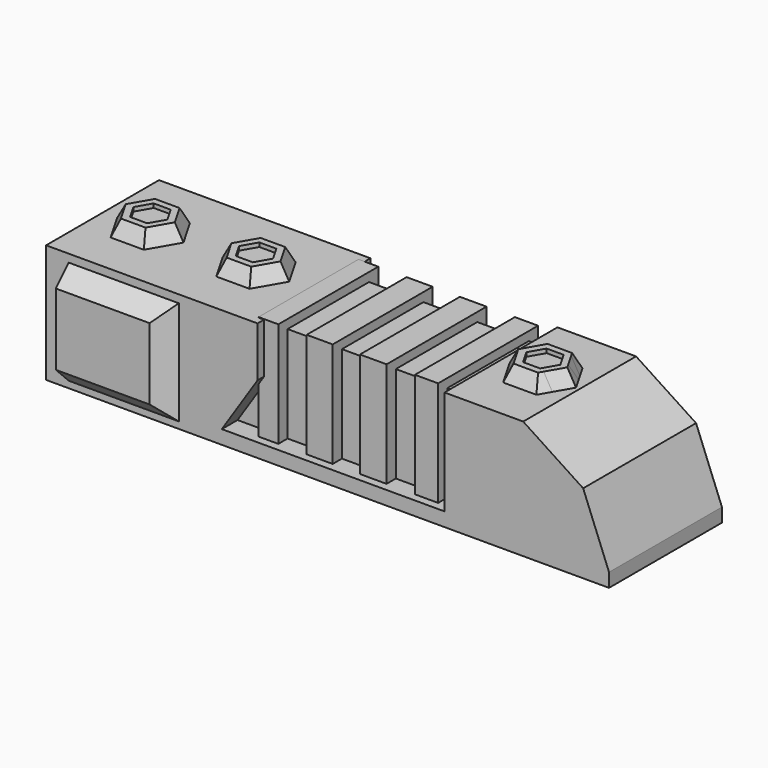
from build123d import *

# Parameters (mm, degrees)
F1_DEPTH      = 15.494
F2_W          = 63.7689922005
F2_H          = 21.1620870978
F3_DEPTH      = 11.176
F4_W          = 5.0933659077
F4_H          = 23.1081098318
F4_W_2        = 5.8479374275
F4_W_3        = 5.7101263665
F4_W_4        = 4.3384544551
F5_DEPTH      = 13.716
F7_DEPTH      = 26.289
F8_T4_DEPTH   = 30.6763762067
F8_T11_DEPTH  = 30.6763762067
F8_T18_DEPTH  = 30.6763762067
F8_T25_DEPTH  = 30.6763762067
F8_T32_DEPTH  = 30.6763762067
F8_T39_DEPTH  = 30.6763762067
F8_T46_DEPTH  = 30.6763762067
F8_T53_DEPTH  = 30.6763762067
F8_T60_DEPTH  = 30.6763762067
F8_T67_DEPTH  = 30.6763762067
F8_T74_DEPTH  = 30.6763762067
F8_T81_DEPTH  = 30.6763762067
F8_T89_DEPTH  = 30.6763762067
F8_T94_DEPTH  = 30.6763762067
F8_T103_DEPTH = 30.6763762067
F8_T109_DEPTH = 30.6763762067
F8_T118_DEPTH = 30.6763762067
F8_T123_DEPTH = 30.6763762067
F8_T131_DEPTH = 30.6763762067
F8_T137_DEPTH = 30.6763762067
F8_T146_DEPTH = 30.6763762067
F8_T152_DEPTH = 30.6763762067
F8_T161_DEPTH = 30.6763762067
F8_T167_DEPTH = 30.6763762067
F8_T175_DEPTH = 30.6763762067
F8_T180_DEPTH = 30.6763762067
F8_T189_DEPTH = 30.6763762067
F8_T195_DEPTH = 30.6763762067
F8_T203_DEPTH = 30.6763762067
F8_T208_DEPTH = 30.6763762067
F8_T216_DEPTH = 30.6763762067
F8_T222_DEPTH = 30.6763762067
F8_T230_DEPTH = 30.6763762067
F8_T236_DEPTH = 30.6763762067
F8_T244_DEPTH = 30.6763762067
F8_T249_DEPTH = 30.6763762067
F10_DEPTH     = 51.054
F11_W         = 19.0685391426
F11_H         = 12.6749693882
F12_DEPTH     = 19.05
F13_T4_DEPTH  = 19.0685391426
F13_T9_DEPTH  = 12.6749693882
F13_T14_DEPTH = 19.0685391426
F13_T19_DEPTH = 19.0685391426
F13_T24_DEPTH = 12.6749693882
F13_T29_DEPTH = 19.0685391426
F13_T35_DEPTH = 32.1326887215
F13_T40_DEPTH = 25.739118967
F13_T49_DEPTH = 32.1326887215
F13_T54_DEPTH = 25.739118967
F13_T63_DEPTH = 32.1326887215
F13_T68_DEPTH = 25.739118967
F13_T77_DEPTH = 32.1326887215
F13_T82_DEPTH = 25.739118967
F14_T4_DEPTH  = 30.6763762067
F14_T11_DEPTH = 30.6763762067
F14_T18_DEPTH = 30.6763762067
F14_T25_DEPTH = 30.6763762067
F14_T32_DEPTH = 30.6763762067
F14_T39_DEPTH = 30.6763762067
F15_DEPTH     = 25.4


# Not quite as in the source:
# - a fillet or chamfer that OpenCascade refuses, or shapes differently, is made with other operations: its cross-section is extruded or revolved along the edge and cut away or added


with BuildPart() as f1:
    # F0 (on Front) → F1 (new body, symmetric)
    with BuildSketch(Plane.XZ):
        Polygon((-61.5085139871, 22.9873508215), (-61.5085139871, 0), (-22.9227617383, 0), (-15.0710064918, 11.9948992506), (-15.0710064918, 22.9873508215), align=None)
        Polygon((-22.9227617383, 0), (-61.5085139871, 0), (-61.5085139871, -3.0355965719), (62.1004961431, -3.0355965719), (62.1004961431, 0), (25.9824357927, 0), align=None)
        Polygon((25.9824357927, 22.9873508215), (25.9824357927, 0), (62.1004961431, 0), (56.4225864728, 14.368809454), (43.256290257, 22.9873508215), align=None)
    extrude(amount=F1_DEPTH, both=True)

    # F2 (on Front) → F3 (join, symmetric)
    with BuildSketch(Plane.XZ):
        with Locations((1.4678305015, 10.5810435489)):
            Rectangle(F2_W, F2_H)
    extrude(amount=F3_DEPTH, both=True)

    # F4 (on Front) → F5 (join, symmetric)
    with BuildSketch(Plane.XZ):
        with Locations((20.6055901945, 11.5540549159)):
            Rectangle(F4_W, F4_H)
        with Locations((8.9097167365, 11.5540549159)):
            Rectangle(F4_W_2, F4_H)
        with Locations((-2.8550631832, 11.5540549159)):
            Rectangle(F4_W_3, F4_H)
        with Locations((-14.1045767814, 11.5540549159)):
            Rectangle(F4_W_4, F4_H)
    extrude(amount=F5_DEPTH, both=True)

    # F6 (on Top) → F7 (join)
    with BuildSketch(Plane.XY):
        Polygon((-48.8487076287, 3.7790879142), (-53.2124224778, 3.7790879142), (-55.3942799023, 0), (-53.2124224778, -3.7790879142), (-48.8487076287, -3.7790879142), (-46.6668502042, 0), align=None)
        Polygon((-25.6386999314, 3.7790879142), (-30.0024147804, 3.7790879142), (-32.1842722049, 0), (-30.0024147804, -3.7790879142), (-25.6386999314, -3.7790879142), (-23.4568425068, 0), align=None)
        Polygon((37.3479384656, 3.7790879142), (32.9842236166, 3.7790879142), (30.802366192, 0), (32.9842236166, -3.7790879142), (37.3479384656, -3.7790879142), (39.5297958902, 0), align=None)
    extrude(amount=F7_DEPTH)

    # F8: chamfer of 5.08 x 2.54 on 12 edges, made by hand


with BuildPart() as f8_tool2:
    # F8_s3 → F8_t4 (new body)
    with BuildSketch(Plane.YZ.offset(-35.6923769499)):
        Polygon((-6.3190879142, 22.9873508215), (-3.7790879142, 28.0673508215), (-3.7790879142, 22.9873508215), align=None)
    extrude(amount=-F8_T4_DEPTH)

    split(bisect_by=Plane(origin=(-41.5457099267, -23.9864268099, 0), x_dir=(0, 0, 1), z_dir=(0.8660254038, 0.5, 0)), keep=Keep.TOP)

    split(bisect_by=Plane(origin=(-35.0001376531, 20.2073388957, 0), x_dir=(0, 0, 1), z_dir=(-0.8660254038, 0.5, 0)), keep=Keep.TOP)

    split(bisect_by=Plane.XY.offset(26.289), keep=Keep.BOTTOM)


with BuildPart() as f1_1:
    add(f1.part)

    # F8_t1: union F8_tool2
    add(f8_tool2.part)


with BuildPart() as f8_tool9:
    # F8_s10 → F8_t11 (new body)
    with BuildSketch(Plane(origin=(-5.0885472116, -8.8136223072, 0), x_dir=(0, 0, 1), z_dir=(-0.5, -0.8660254038, 0))):
        Polygon((22.9873508215, 37.8746777914), (28.0673508215, 40.4146777914), (22.9873508215, 40.4146777914), align=None)
    extrude(amount=F8_T11_DEPTH)

    split(bisect_by=Plane.XZ.offset(3.7790879142), keep=Keep.BOTTOM)

    split(bisect_by=Plane(origin=(-35.0001376531, -20.2073388957, 0), x_dir=(0, 0, 1), z_dir=(-0.8660254038, -0.5, 0)), keep=Keep.TOP)

    split(bisect_by=Plane.XY.offset(26.289), keep=Keep.BOTTOM)


with BuildPart() as f1_2:
    add(f1_1.part)

    # F8_t8: union F8_tool9
    add(f8_tool9.part)


with BuildPart() as f8_tool16:
    # F8_s17 → F8_t18 (new body)
    with BuildSketch(Plane(origin=(-5.0885472116, 8.8136223072, 0), x_dir=(0, 0, 1), z_dir=(-0.5, 0.8660254038, 0))):
        Polygon((22.9873508215, -50.5128536197), (28.0673508215, -47.9728536197), (22.9873508215, -47.9728536197), align=None)
    extrude(amount=F8_T18_DEPTH)

    split(bisect_by=Plane(origin=(-41.5457099267, 23.9864268099, 0), x_dir=(0, 0, 1), z_dir=(0.8660254038, -0.5, 0)), keep=Keep.TOP)

    split(bisect_by=Plane.XZ.offset(3.7790879142), keep=Keep.BOTTOM)

    split(bisect_by=Plane.XY.offset(26.289), keep=Keep.BOTTOM)


with BuildPart() as f1_3:
    add(f1_2.part)

    # F8_t15: union F8_tool16
    add(f8_tool16.part)


with BuildPart() as f8_tool23:
    # F8_s24 → F8_t25 (new body)
    with BuildSketch(Plane.YZ.offset(-66.3687531566)):
        Polygon((6.3190879142, 22.9873508215), (3.7790879142, 28.0673508215), (3.7790879142, 22.9873508215), align=None)
    extrude(amount=F8_T25_DEPTH)

    split(bisect_by=Plane(origin=(-41.5457099267, 23.9864268099, 0), x_dir=(0, 0, 1), z_dir=(0.8660254038, -0.5, 0)), keep=Keep.TOP)

    split(bisect_by=Plane(origin=(-35.0001376531, -20.2073388957, 0), x_dir=(0, 0, 1), z_dir=(-0.8660254038, -0.5, 0)), keep=Keep.TOP)

    split(bisect_by=Plane.XY.offset(26.289), keep=Keep.BOTTOM)


with BuildPart() as f1_4:
    add(f1_3.part)

    # F8_t22: union F8_tool23
    add(f8_tool23.part)


with BuildPart() as f8_tool30:
    # F8_s31 → F8_t32 (new body)
    with BuildSketch(Plane(origin=(-20.426735315, 35.3801433983, 0), x_dir=(0, 0, 1), z_dir=(0.5, -0.8660254038, 0))):
        Polygon((22.9873508215, 37.8746777914), (28.0673508215, 40.4146777914), (22.9873508215, 40.4146777914), align=None)
    extrude(amount=F8_T32_DEPTH)

    split(bisect_by=Plane(origin=(-35.0001376531, 20.2073388957, 0), x_dir=(0, 0, 1), z_dir=(-0.8660254038, 0.5, 0)), keep=Keep.TOP)

    split(bisect_by=Plane.XZ.offset(-3.7790879142), keep=Keep.TOP)

    split(bisect_by=Plane.XY.offset(26.289), keep=Keep.BOTTOM)


with BuildPart() as f1_5:
    add(f1_4.part)

    # F8_t29: union F8_tool30
    add(f8_tool30.part)


with BuildPart() as f8_tool37:
    # F8_s38 → F8_t39 (new body)
    with BuildSketch(Plane.YZ.offset(-12.4823692525)):
        Polygon((-6.3190879142, 22.9873508215), (-3.7790879142, 28.0673508215), (-3.7790879142, 22.9873508215), align=None)
    extrude(amount=-F8_T39_DEPTH)

    split(bisect_by=Plane(origin=(-24.1382041537, -13.9361986659, 0), x_dir=(0, 0, 1), z_dir=(0.8660254038, 0.5, 0)), keep=Keep.TOP)

    split(bisect_by=Plane(origin=(-17.5926318801, 10.1571107517, 0), x_dir=(0, 0, 1), z_dir=(-0.8660254038, 0.5, 0)), keep=Keep.TOP)

    split(bisect_by=Plane.XY.offset(26.289), keep=Keep.BOTTOM)


with BuildPart() as f1_6:
    add(f1_5.part)

    # F8_t36: union F8_tool37
    add(f8_tool37.part)


with BuildPart() as f8_tool44:
    # F8_s45 → F8_t46 (new body)
    with BuildSketch(Plane(origin=(0.7139547127, -1.2366058367, 0), x_dir=(0, 0, 1), z_dir=(-0.5, 0.8660254038, 0))):
        Polygon((22.9873508215, -30.4123973318), (28.0673508215, -27.8723973318), (22.9873508215, -27.8723973318), align=None)
    extrude(amount=F8_T46_DEPTH)

    split(bisect_by=Plane(origin=(-24.1382041537, 13.9361986659, 0), x_dir=(0, 0, 1), z_dir=(0.8660254038, -0.5, 0)), keep=Keep.TOP)

    split(bisect_by=Plane.XZ.offset(3.7790879142), keep=Keep.BOTTOM)

    split(bisect_by=Plane.XY.offset(26.289), keep=Keep.BOTTOM)


with BuildPart() as f1_7:
    add(f1_6.part)

    # F8_t43: union F8_tool44
    add(f8_tool44.part)


with BuildPart() as f8_tool51:
    # F8_s52 → F8_t53 (new body)
    with BuildSketch(Plane(origin=(-14.6242333907, -25.3299152544, 0), x_dir=(0, 0, 1), z_dir=(0.5, 0.8660254038, 0))):
        Polygon((22.9873508215, -30.4123973318), (28.0673508215, -27.8723973318), (22.9873508215, -27.8723973318), align=None)
    extrude(amount=F8_T53_DEPTH)

    split(bisect_by=Plane(origin=(-24.1382041537, -13.9361986659, 0), x_dir=(0, 0, 1), z_dir=(0.8660254038, 0.5, 0)), keep=Keep.TOP)

    split(bisect_by=Plane.XY.offset(26.289), keep=Keep.BOTTOM)

    split(bisect_by=Plane.XZ.offset(-3.7790879142), keep=Keep.TOP)


with BuildPart() as f1_8:
    add(f1_7.part)

    # F8_t50: union F8_tool51
    add(f8_tool51.part)


with BuildPart() as f8_tool58:
    # F8_s59 → F8_t60 (new body)
    with BuildSketch(Plane.YZ.offset(-43.1587454592)):
        Polygon((6.3190879142, 22.9873508215), (3.7790879142, 28.0673508215), (3.7790879142, 22.9873508215), align=None)
    extrude(amount=F8_T60_DEPTH)

    split(bisect_by=Plane(origin=(-24.1382041537, 13.9361986659, 0), x_dir=(0, 0, 1), z_dir=(0.8660254038, -0.5, 0)), keep=Keep.TOP)

    split(bisect_by=Plane(origin=(-17.5926318801, -10.1571107517, 0), x_dir=(0, 0, 1), z_dir=(-0.8660254038, -0.5, 0)), keep=Keep.TOP)

    split(bisect_by=Plane.XY.offset(26.289), keep=Keep.BOTTOM)


with BuildPart() as f1_9:
    add(f1_8.part)

    # F8_t57: union F8_tool58
    add(f8_tool58.part)


with BuildPart() as f8_tool65:
    # F8_s66 → F8_t67 (new body)
    with BuildSketch(Plane(origin=(-14.6242333907, 25.3299152544, 0), x_dir=(0, 0, 1), z_dir=(0.5, -0.8660254038, 0))):
        Polygon((22.9873508215, 17.7742215035), (28.0673508215, 20.3142215035), (22.9873508215, 20.3142215035), align=None)
    extrude(amount=F8_T67_DEPTH)

    split(bisect_by=Plane(origin=(-17.5926318801, 10.1571107517, 0), x_dir=(0, 0, 1), z_dir=(-0.8660254038, 0.5, 0)), keep=Keep.TOP)

    split(bisect_by=Plane.XZ.offset(-3.7790879142), keep=Keep.TOP)

    split(bisect_by=Plane.XY.offset(26.289), keep=Keep.BOTTOM)


with BuildPart() as f1_10:
    add(f1_9.part)

    # F8_t64: union F8_tool65
    add(f8_tool65.part)


with BuildPart() as f8_tool72:
    # F8_s73 → F8_t74 (new body)
    with BuildSketch(Plane(origin=(0.7139547127, 1.2366058367, 0), x_dir=(0, 0, 1), z_dir=(-0.5, -0.8660254038, 0))):
        Polygon((22.9873508215, 17.7742215035), (28.0673508215, 20.3142215035), (22.9873508215, 20.3142215035), align=None)
    extrude(amount=F8_T74_DEPTH)

    split(bisect_by=Plane.XZ.offset(3.7790879142), keep=Keep.BOTTOM)

    split(bisect_by=Plane(origin=(-17.5926318801, -10.1571107517, 0), x_dir=(0, 0, 1), z_dir=(-0.8660254038, -0.5, 0)), keep=Keep.TOP)

    split(bisect_by=Plane.XY.offset(26.289), keep=Keep.BOTTOM)


with BuildPart() as f1_11:
    add(f1_10.part)

    # F8_t71: union F8_tool72
    add(f8_tool72.part)


with BuildPart() as f8_tool79:
    # F8_s80 → F8_t81 (new body)
    with BuildSketch(Plane(origin=(-20.426735315, -35.3801433983, 0), x_dir=(0, 0, 1), z_dir=(0.5, 0.8660254038, 0))):
        Polygon((22.9873508215, -50.5128536197), (28.0673508215, -47.9728536197), (22.9873508215, -47.9728536197), align=None)
    extrude(amount=F8_T81_DEPTH)

    split(bisect_by=Plane(origin=(-41.5457099267, -23.9864268099, 0), x_dir=(0, 0, 1), z_dir=(0.8660254038, 0.5, 0)), keep=Keep.TOP)

    split(bisect_by=Plane.XY.offset(26.289), keep=Keep.BOTTOM)

    split(bisect_by=Plane.XZ.offset(-3.7790879142), keep=Keep.TOP)


with BuildPart() as f1_12:
    add(f1_11.part)

    # F8_t78: union F8_tool79
    add(f8_tool79.part)


with BuildPart() as f8_tool87:
    # F8_s88 → F8_t89 (new body)
    with BuildSketch(Plane.YZ.offset(-35.6923769499)):
        Polygon((-6.3190879142, 22.9873508215), (-3.7790879142, 28.0673508215), (-3.7790879142, 22.9873508215), align=None)
    extrude(amount=-F8_T89_DEPTH)

    split(bisect_by=Plane(origin=(-35.0001376531, 20.2073388957, 0), x_dir=(0, 0, 1), z_dir=(0.8660254038, -0.5, 0)), keep=Keep.TOP)

    split(bisect_by=Plane.XY.offset(26.289), keep=Keep.BOTTOM)


with BuildPart() as f8_tool92:
    # F8_s93 → F8_t94 (new body)
    with BuildSketch(Plane(origin=(-5.0885472116, -8.8136223072, 0), x_dir=(0, 0, 1), z_dir=(-0.5, -0.8660254038, 0))):
        Polygon((22.9873508215, 37.8746777914), (28.0673508215, 40.4146777914), (22.9873508215, 40.4146777914), align=None)
    extrude(amount=F8_T94_DEPTH)

    split(bisect_by=Plane.XZ.offset(15.494), keep=Keep.BOTTOM)

    split(bisect_by=Plane.XZ.offset(3.7790879142), keep=Keep.TOP)

    split(bisect_by=Plane.XY.offset(26.289), keep=Keep.BOTTOM)


with BuildPart() as f8_tool87_1:
    add(f8_tool87.part)

    # F8_t98: intersect F8_tool92
    add(f8_tool92.part, mode=Mode.INTERSECT)


with BuildPart() as f1_13:
    add(f1_12.part)

    # F8_t85: union F8_tool87
    add(f8_tool87_1.part)


with BuildPart() as f8_tool101:
    # F8_s102 → F8_t103 (new body)
    with BuildSketch(Plane(origin=(-5.0885472116, 8.8136223072, 0), x_dir=(0, 0, 1), z_dir=(-0.5, 0.8660254038, 0))):
        Polygon((22.9873508215, -50.5128536197), (28.0673508215, -47.9728536197), (22.9873508215, -47.9728536197), align=None)
    extrude(amount=F8_T103_DEPTH)

    split(bisect_by=Plane.XZ.offset(15.494), keep=Keep.BOTTOM)

    split(bisect_by=Plane.XZ.offset(3.7790879142), keep=Keep.TOP)

    split(bisect_by=Plane.XY.offset(26.289), keep=Keep.BOTTOM)


with BuildPart() as f8_tool107:
    # F8_s108 → F8_t109 (new body)
    with BuildSketch(Plane.YZ.offset(-35.6923769499)):
        Polygon((-6.3190879142, 22.9873508215), (-3.7790879142, 28.0673508215), (-3.7790879142, 22.9873508215), align=None)
    extrude(amount=-F8_T109_DEPTH)

    split(bisect_by=Plane.YZ.offset(-61.5085139871), keep=Keep.TOP)

    split(bisect_by=Plane(origin=(-41.5457099267, -23.9864268099, 0), x_dir=(0, 0, 1), z_dir=(-0.8660254038, -0.5, 0)), keep=Keep.TOP)

    split(bisect_by=Plane.XY.offset(26.289), keep=Keep.BOTTOM)


with BuildPart() as f8_tool101_1:
    add(f8_tool101.part)

    # F8_t113: intersect F8_tool107
    add(f8_tool107.part, mode=Mode.INTERSECT)


with BuildPart() as f1_14:
    add(f1_13.part)

    # F8_t99: union F8_tool101
    add(f8_tool101_1.part)


with BuildPart() as f8_tool116:
    # F8_s117 → F8_t118 (new body)
    with BuildSketch(Plane(origin=(-5.0885472116, -8.8136223072, 0), x_dir=(0, 0, 1), z_dir=(-0.5, -0.8660254038, 0))):
        Polygon((22.9873508215, 37.8746777914), (28.0673508215, 40.4146777914), (22.9873508215, 40.4146777914), align=None)
    extrude(amount=F8_T118_DEPTH)

    split(bisect_by=Plane(origin=(-35.0001376531, -20.2073388957, 0), x_dir=(0, 0, 1), z_dir=(0.8660254038, 0.5, 0)), keep=Keep.TOP)

    split(bisect_by=Plane.XY.offset(26.289), keep=Keep.BOTTOM)


with BuildPart() as f8_tool121:
    # F8_s122 → F8_t123 (new body)
    with BuildSketch(Plane(origin=(-20.426735315, 35.3801433983, 0), x_dir=(0, 0, 1), z_dir=(0.5, -0.8660254038, 0))):
        Polygon((22.9873508215, 37.8746777914), (28.0673508215, 40.4146777914), (22.9873508215, 40.4146777914), align=None)
    extrude(amount=F8_T123_DEPTH)

    split(bisect_by=Plane(origin=(-35.0001376531, 20.2073388957, 0), x_dir=(0, 0, 1), z_dir=(0.8660254038, -0.5, 0)), keep=Keep.TOP)

    split(bisect_by=Plane.XY.offset(26.289), keep=Keep.BOTTOM)


with BuildPart() as f8_tool116_1:
    add(f8_tool116.part)

    # F8_t126: intersect F8_tool121
    add(f8_tool121.part, mode=Mode.INTERSECT)


with BuildPart() as f1_15:
    add(f1_14.part)

    # F8_t114: union F8_tool116
    add(f8_tool116_1.part)


with BuildPart() as f8_tool129:
    # F8_s130 → F8_t131 (new body)
    with BuildSketch(Plane(origin=(-20.426735315, -35.3801433983, 0), x_dir=(0, 0, 1), z_dir=(0.5, 0.8660254038, 0))):
        Polygon((22.9873508215, -50.5128536197), (28.0673508215, -47.9728536197), (22.9873508215, -47.9728536197), align=None)
    extrude(amount=F8_T131_DEPTH)

    split(bisect_by=Plane.YZ.offset(-61.5085139871), keep=Keep.TOP)

    split(bisect_by=Plane(origin=(-41.5457099267, -23.9864268099, 0), x_dir=(0, 0, 1), z_dir=(-0.8660254038, -0.5, 0)), keep=Keep.TOP)

    split(bisect_by=Plane.XY.offset(26.289), keep=Keep.BOTTOM)


with BuildPart() as f8_tool135:
    # F8_s136 → F8_t137 (new body)
    with BuildSketch(Plane(origin=(-5.0885472116, 8.8136223072, 0), x_dir=(0, 0, 1), z_dir=(-0.5, 0.8660254038, 0))):
        Polygon((22.9873508215, -50.5128536197), (28.0673508215, -47.9728536197), (22.9873508215, -47.9728536197), align=None)
    extrude(amount=F8_T137_DEPTH)

    split(bisect_by=Plane.YZ.offset(-61.5085139871), keep=Keep.TOP)

    split(bisect_by=Plane(origin=(-41.5457099267, 23.9864268099, 0), x_dir=(0, 0, 1), z_dir=(-0.8660254038, 0.5, 0)), keep=Keep.TOP)

    split(bisect_by=Plane.XY.offset(26.289), keep=Keep.BOTTOM)


with BuildPart() as f8_tool129_1:
    add(f8_tool129.part)

    # F8_t141: intersect F8_tool135
    add(f8_tool135.part, mode=Mode.INTERSECT)


with BuildPart() as f1_16:
    add(f1_15.part)

    # F8_t127: union F8_tool129
    add(f8_tool129_1.part)


with BuildPart() as f8_tool144:
    # F8_s145 → F8_t146 (new body)
    with BuildSketch(Plane(origin=(-20.426735315, -35.3801433983, 0), x_dir=(0, 0, 1), z_dir=(0.5, 0.8660254038, 0))):
        Polygon((22.9873508215, -50.5128536197), (28.0673508215, -47.9728536197), (22.9873508215, -47.9728536197), align=None)
    extrude(amount=F8_T146_DEPTH)

    split(bisect_by=Plane.XZ.offset(-15.494), keep=Keep.TOP)

    split(bisect_by=Plane.XY.offset(26.289), keep=Keep.BOTTOM)

    split(bisect_by=Plane.XZ.offset(-3.7790879142), keep=Keep.BOTTOM)


with BuildPart() as f8_tool150:
    # F8_s151 → F8_t152 (new body)
    with BuildSketch(Plane.YZ.offset(-66.3687531566)):
        Polygon((6.3190879142, 22.9873508215), (3.7790879142, 28.0673508215), (3.7790879142, 22.9873508215), align=None)
    extrude(amount=F8_T152_DEPTH)

    split(bisect_by=Plane.YZ.offset(-61.5085139871), keep=Keep.TOP)

    split(bisect_by=Plane(origin=(-41.5457099267, 23.9864268099, 0), x_dir=(0, 0, 1), z_dir=(-0.8660254038, 0.5, 0)), keep=Keep.TOP)

    split(bisect_by=Plane.XY.offset(26.289), keep=Keep.BOTTOM)


with BuildPart() as f8_tool144_1:
    add(f8_tool144.part)

    # F8_t156: intersect F8_tool150
    add(f8_tool150.part, mode=Mode.INTERSECT)


with BuildPart() as f1_17:
    add(f1_16.part)

    # F8_t142: union F8_tool144
    add(f8_tool144_1.part)


with BuildPart() as f8_tool159:
    # F8_s160 → F8_t161 (new body)
    with BuildSketch(Plane(origin=(-20.426735315, 35.3801433983, 0), x_dir=(0, 0, 1), z_dir=(0.5, -0.8660254038, 0))):
        Polygon((22.9873508215, 37.8746777914), (28.0673508215, 40.4146777914), (22.9873508215, 40.4146777914), align=None)
    extrude(amount=F8_T161_DEPTH)

    split(bisect_by=Plane.XZ.offset(-15.494), keep=Keep.TOP)

    split(bisect_by=Plane.XZ.offset(-3.7790879142), keep=Keep.BOTTOM)

    split(bisect_by=Plane.XY.offset(26.289), keep=Keep.BOTTOM)


with BuildPart() as f8_tool165:
    # F8_s166 → F8_t167 (new body)
    with BuildSketch(Plane.YZ.offset(-66.3687531566)):
        Polygon((6.3190879142, 22.9873508215), (3.7790879142, 28.0673508215), (3.7790879142, 22.9873508215), align=None)
    extrude(amount=F8_T167_DEPTH)

    split(bisect_by=Plane(origin=(-35.0001376531, -20.2073388957, 0), x_dir=(0, 0, 1), z_dir=(0.8660254038, 0.5, 0)), keep=Keep.TOP)

    split(bisect_by=Plane.XY.offset(26.289), keep=Keep.BOTTOM)


with BuildPart() as f8_tool159_1:
    add(f8_tool159.part)

    # F8_t170: intersect F8_tool165
    add(f8_tool165.part, mode=Mode.INTERSECT)


with BuildPart() as f1_18:
    add(f1_17.part)

    # F8_t157: union F8_tool159
    add(f8_tool159_1.part)


with BuildPart() as f8_tool173:
    # F8_s174 → F8_t175 (new body)
    with BuildSketch(Plane.YZ.offset(-12.4823692525)):
        Polygon((-6.3190879142, 22.9873508215), (-3.7790879142, 28.0673508215), (-3.7790879142, 22.9873508215), align=None)
    extrude(amount=-F8_T175_DEPTH)

    split(bisect_by=Plane(origin=(-17.5926318801, 10.1571107517, 0), x_dir=(0, 0, 1), z_dir=(0.8660254038, -0.5, 0)), keep=Keep.TOP)

    split(bisect_by=Plane.XY.offset(26.289), keep=Keep.BOTTOM)


with BuildPart() as f8_tool178:
    # F8_s179 → F8_t180 (new body)
    with BuildSketch(Plane(origin=(0.7139547127, 1.2366058367, 0), x_dir=(0, 0, 1), z_dir=(-0.5, -0.8660254038, 0))):
        Polygon((22.9873508215, 17.7742215035), (28.0673508215, 20.3142215035), (22.9873508215, 20.3142215035), align=None)
    extrude(amount=F8_T180_DEPTH)

    split(bisect_by=Plane.XZ.offset(15.494), keep=Keep.BOTTOM)

    split(bisect_by=Plane.XZ.offset(3.7790879142), keep=Keep.TOP)

    split(bisect_by=Plane.XY.offset(26.289), keep=Keep.BOTTOM)


with BuildPart() as f8_tool173_1:
    add(f8_tool173.part)

    # F8_t184: intersect F8_tool178
    add(f8_tool178.part, mode=Mode.INTERSECT)


with BuildPart() as f1_19:
    add(f1_18.part)

    # F8_t171: union F8_tool173
    add(f8_tool173_1.part)


with BuildPart() as f8_tool187:
    # F8_s188 → F8_t189 (new body)
    with BuildSketch(Plane(origin=(0.7139547127, -1.2366058367, 0), x_dir=(0, 0, 1), z_dir=(-0.5, 0.8660254038, 0))):
        Polygon((22.9873508215, -30.4123973318), (28.0673508215, -27.8723973318), (22.9873508215, -27.8723973318), align=None)
    extrude(amount=F8_T189_DEPTH)

    split(bisect_by=Plane.XZ.offset(15.494), keep=Keep.BOTTOM)

    split(bisect_by=Plane.XZ.offset(3.7790879142), keep=Keep.TOP)

    split(bisect_by=Plane.XY.offset(26.289), keep=Keep.BOTTOM)


with BuildPart() as f8_tool193:
    # F8_s194 → F8_t195 (new body)
    with BuildSketch(Plane.YZ.offset(-12.4823692525)):
        Polygon((-6.3190879142, 22.9873508215), (-3.7790879142, 28.0673508215), (-3.7790879142, 22.9873508215), align=None)
    extrude(amount=-F8_T195_DEPTH)

    split(bisect_by=Plane(origin=(-24.1382041537, -13.9361986659, 0), x_dir=(0, 0, 1), z_dir=(-0.8660254038, -0.5, 0)), keep=Keep.TOP)

    split(bisect_by=Plane.XY.offset(26.289), keep=Keep.BOTTOM)


with BuildPart() as f8_tool187_1:
    add(f8_tool187.part)

    # F8_t198: intersect F8_tool193
    add(f8_tool193.part, mode=Mode.INTERSECT)


with BuildPart() as f1_20:
    add(f1_19.part)

    # F8_t185: union F8_tool187
    add(f8_tool187_1.part)


with BuildPart() as f8_tool201:
    # F8_s202 → F8_t203 (new body)
    with BuildSketch(Plane(origin=(-14.6242333907, -25.3299152544, 0), x_dir=(0, 0, 1), z_dir=(0.5, 0.8660254038, 0))):
        Polygon((22.9873508215, -30.4123973318), (28.0673508215, -27.8723973318), (22.9873508215, -27.8723973318), align=None)
    extrude(amount=F8_T203_DEPTH)

    split(bisect_by=Plane(origin=(-24.1382041537, -13.9361986659, 0), x_dir=(0, 0, 1), z_dir=(-0.8660254038, -0.5, 0)), keep=Keep.TOP)

    split(bisect_by=Plane.XY.offset(26.289), keep=Keep.BOTTOM)


with BuildPart() as f8_tool206:
    # F8_s207 → F8_t208 (new body)
    with BuildSketch(Plane(origin=(0.7139547127, -1.2366058367, 0), x_dir=(0, 0, 1), z_dir=(-0.5, 0.8660254038, 0))):
        Polygon((22.9873508215, -30.4123973318), (28.0673508215, -27.8723973318), (22.9873508215, -27.8723973318), align=None)
    extrude(amount=F8_T208_DEPTH)

    split(bisect_by=Plane(origin=(-24.1382041537, 13.9361986659, 0), x_dir=(0, 0, 1), z_dir=(-0.8660254038, 0.5, 0)), keep=Keep.TOP)

    split(bisect_by=Plane.XY.offset(26.289), keep=Keep.BOTTOM)


with BuildPart() as f8_tool201_1:
    add(f8_tool201.part)

    # F8_t211: intersect F8_tool206
    add(f8_tool206.part, mode=Mode.INTERSECT)


with BuildPart() as f1_21:
    add(f1_20.part)

    # F8_t199: union F8_tool201
    add(f8_tool201_1.part)


with BuildPart() as f8_tool214:
    # F8_s215 → F8_t216 (new body)
    with BuildSketch(Plane(origin=(-14.6242333907, -25.3299152544, 0), x_dir=(0, 0, 1), z_dir=(0.5, 0.8660254038, 0))):
        Polygon((22.9873508215, -30.4123973318), (28.0673508215, -27.8723973318), (22.9873508215, -27.8723973318), align=None)
    extrude(amount=F8_T216_DEPTH)

    split(bisect_by=Plane.XZ.offset(-15.494), keep=Keep.TOP)

    split(bisect_by=Plane.XY.offset(26.289), keep=Keep.BOTTOM)

    split(bisect_by=Plane.XZ.offset(-3.7790879142), keep=Keep.BOTTOM)


with BuildPart() as f8_tool220:
    # F8_s221 → F8_t222 (new body)
    with BuildSketch(Plane.YZ.offset(-43.1587454592)):
        Polygon((6.3190879142, 22.9873508215), (3.7790879142, 28.0673508215), (3.7790879142, 22.9873508215), align=None)
    extrude(amount=F8_T222_DEPTH)

    split(bisect_by=Plane(origin=(-24.1382041537, 13.9361986659, 0), x_dir=(0, 0, 1), z_dir=(-0.8660254038, 0.5, 0)), keep=Keep.TOP)

    split(bisect_by=Plane.XY.offset(26.289), keep=Keep.BOTTOM)


with BuildPart() as f8_tool214_1:
    add(f8_tool214.part)

    # F8_t225: intersect F8_tool220
    add(f8_tool220.part, mode=Mode.INTERSECT)


with BuildPart() as f1_22:
    add(f1_21.part)

    # F8_t212: union F8_tool214
    add(f8_tool214_1.part)


with BuildPart() as f8_tool228:
    # F8_s229 → F8_t230 (new body)
    with BuildSketch(Plane(origin=(-14.6242333907, 25.3299152544, 0), x_dir=(0, 0, 1), z_dir=(0.5, -0.8660254038, 0))):
        Polygon((22.9873508215, 17.7742215035), (28.0673508215, 20.3142215035), (22.9873508215, 20.3142215035), align=None)
    extrude(amount=F8_T230_DEPTH)

    split(bisect_by=Plane.XZ.offset(-15.494), keep=Keep.TOP)

    split(bisect_by=Plane.XZ.offset(-3.7790879142), keep=Keep.BOTTOM)

    split(bisect_by=Plane.XY.offset(26.289), keep=Keep.BOTTOM)


with BuildPart() as f8_tool234:
    # F8_s235 → F8_t236 (new body)
    with BuildSketch(Plane.YZ.offset(-43.1587454592)):
        Polygon((6.3190879142, 22.9873508215), (3.7790879142, 28.0673508215), (3.7790879142, 22.9873508215), align=None)
    extrude(amount=F8_T236_DEPTH)

    split(bisect_by=Plane(origin=(-17.5926318801, -10.1571107517, 0), x_dir=(0, 0, 1), z_dir=(0.8660254038, 0.5, 0)), keep=Keep.TOP)

    split(bisect_by=Plane.XY.offset(26.289), keep=Keep.BOTTOM)


with BuildPart() as f8_tool228_1:
    add(f8_tool228.part)

    # F8_t239: intersect F8_tool234
    add(f8_tool234.part, mode=Mode.INTERSECT)


with BuildPart() as f1_23:
    add(f1_22.part)

    # F8_t226: union F8_tool228
    add(f8_tool228_1.part)


with BuildPart() as f8_tool242:
    # F8_s243 → F8_t244 (new body)
    with BuildSketch(Plane(origin=(0.7139547127, 1.2366058367, 0), x_dir=(0, 0, 1), z_dir=(-0.5, -0.8660254038, 0))):
        Polygon((22.9873508215, 17.7742215035), (28.0673508215, 20.3142215035), (22.9873508215, 20.3142215035), align=None)
    extrude(amount=F8_T244_DEPTH)

    split(bisect_by=Plane(origin=(-17.5926318801, -10.1571107517, 0), x_dir=(0, 0, 1), z_dir=(0.8660254038, 0.5, 0)), keep=Keep.TOP)

    split(bisect_by=Plane.XY.offset(26.289), keep=Keep.BOTTOM)


with BuildPart() as f8_tool247:
    # F8_s248 → F8_t249 (new body)
    with BuildSketch(Plane(origin=(-14.6242333907, 25.3299152544, 0), x_dir=(0, 0, 1), z_dir=(0.5, -0.8660254038, 0))):
        Polygon((22.9873508215, 17.7742215035), (28.0673508215, 20.3142215035), (22.9873508215, 20.3142215035), align=None)
    extrude(amount=F8_T249_DEPTH)

    split(bisect_by=Plane(origin=(-17.5926318801, 10.1571107517, 0), x_dir=(0, 0, 1), z_dir=(0.8660254038, -0.5, 0)), keep=Keep.TOP)

    split(bisect_by=Plane.XY.offset(26.289), keep=Keep.BOTTOM)


with BuildPart() as f8_tool242_1:
    add(f8_tool242.part)

    # F8_t252: intersect F8_tool247
    add(f8_tool247.part, mode=Mode.INTERSECT)


with BuildPart() as f1_24:
    add(f1_23.part)

    # F8_t240: union F8_tool242
    add(f8_tool242_1.part)

    # F9 (on Top) → F10 (cut)
    with BuildSketch(Plane.XY):
        Polygon((-49.1261490187, 3.2342278864), (-52.8607137004, 3.2342278864), (-54.7279960412, 0), (-52.8607137004, -3.2342278864), (-49.1261490187, -3.2342278864), (-47.2588666778, 0), align=None)
        Polygon((-25.9230461469, 3.2342278864), (-29.6576108286, 3.2342278864), (-31.5248931694, 0), (-29.6576108286, -3.2342278864), (-25.9230461469, -3.2342278864), (-24.0557638061, 0), align=None)
        Polygon((37.1587939063, 3.2342278864), (33.4242292246, 3.2342278864), (31.5569468838, 0), (33.4242292246, -3.2342278864), (37.1587939063, -3.2342278864), (39.0260762471, 0), align=None)
    extrude(amount=F10_DEPTH, mode=Mode.SUBTRACT)

    # F11 (on Front) → F12 (join, symmetric)
    with BuildSketch(Plane.XZ):
        with Locations((-46.9861701131, 9.8413374508)):
            Rectangle(F11_W, F11_H)
    extrude(amount=F12_DEPTH, both=True)

    # F13: chamfer of 5.08 on 6 edges, made by hand


with BuildPart() as f13_tool2:
    # F13_s3 → F13_t4 (new body)
    with BuildSketch(Plane.YZ.offset(-56.5204396844)):
        Polygon((-15.494, -1.5761472433), (-20.574, 3.5038527567), (-15.494, 3.5038527567), align=None)
    extrude(amount=F13_T4_DEPTH)

    split(bisect_by=Plane.XZ.offset(19.05), keep=Keep.BOTTOM)


with BuildPart() as f1_25:
    add(f1_24.part)

    # F13_t1: union F13_tool2
    add(f13_tool2.part)


with BuildPart() as f13_tool7:
    # F13_s8 → F13_t9 (new body)
    with BuildSketch(Plane.XY.offset(3.5038527567)):
        Polygon((-32.3719005418, -15.494), (-37.4519005418, -20.574), (-37.4519005418, -15.494), align=None)
    extrude(amount=F13_T9_DEPTH)

    split(bisect_by=Plane.XZ.offset(19.05), keep=Keep.BOTTOM)


with BuildPart() as f1_26:
    add(f1_25.part)

    # F13_t6: union F13_tool7
    add(f13_tool7.part)


with BuildPart() as f13_tool12:
    # F13_s13 → F13_t14 (new body)
    with BuildSketch(Plane.YZ.offset(-37.4519005418)):
        Polygon((-15.494, 21.2588221449), (-20.574, 16.1788221449), (-15.494, 16.1788221449), align=None)
    extrude(amount=-F13_T14_DEPTH)

    split(bisect_by=Plane.XZ.offset(19.05), keep=Keep.BOTTOM)


with BuildPart() as f1_27:
    add(f1_26.part)

    # F13_t11: union F13_tool12
    add(f13_tool12.part)


with BuildPart() as f13_tool17:
    # F13_s18 → F13_t19 (new body)
    with BuildSketch(Plane.YZ.offset(-56.5204396844)):
        Polygon((15.494, -1.5761472433), (20.574, 3.5038527567), (15.494, 3.5038527567), align=None)
    extrude(amount=F13_T19_DEPTH)

    split(bisect_by=Plane.XZ.offset(-19.05), keep=Keep.TOP)


with BuildPart() as f1_28:
    add(f1_27.part)

    # F13_t16: union F13_tool17
    add(f13_tool17.part)


with BuildPart() as f13_tool22:
    # F13_s23 → F13_t24 (new body)
    with BuildSketch(Plane.XY.offset(3.5038527567)):
        Polygon((-32.3719005418, 15.494), (-37.4519005418, 20.574), (-37.4519005418, 15.494), align=None)
    extrude(amount=F13_T24_DEPTH)

    split(bisect_by=Plane.XZ.offset(-19.05), keep=Keep.TOP)


with BuildPart() as f1_29:
    add(f1_28.part)

    # F13_t21: union F13_tool22
    add(f13_tool22.part)


with BuildPart() as f13_tool27:
    # F13_s28 → F13_t29 (new body)
    with BuildSketch(Plane.YZ.offset(-37.4519005418)):
        Polygon((15.494, 21.2588221449), (20.574, 16.1788221449), (15.494, 16.1788221449), align=None)
    extrude(amount=-F13_T29_DEPTH)

    split(bisect_by=Plane.XZ.offset(-19.05), keep=Keep.TOP)


with BuildPart() as f1_30:
    add(f1_29.part)

    # F13_t26: union F13_tool27
    add(f13_tool27.part)


with BuildPart() as f13_tool33:
    # F13_s34 → F13_t35 (new body)
    with BuildSketch(Plane.YZ.offset(-56.5204396844)):
        Polygon((-15.494, -1.5761472433), (-20.574, 3.5038527567), (-15.494, 3.5038527567), align=None)
    extrude(amount=F13_T35_DEPTH)

    split(bisect_by=Plane.XZ.offset(19.05), keep=Keep.BOTTOM)

    split(bisect_by=Plane.YZ.offset(-37.4519005418), keep=Keep.TOP)


with BuildPart() as f13_tool38:
    # F13_s39 → F13_t40 (new body)
    with BuildSketch(Plane.XY.offset(-9.5602968222)):
        Polygon((-32.3719005418, -15.494), (-37.4519005418, -20.574), (-37.4519005418, -15.494), align=None)
    extrude(amount=F13_T40_DEPTH)

    split(bisect_by=Plane.XY.offset(-3.0355965719), keep=Keep.TOP)

    split(bisect_by=Plane.XY.offset(3.5038527567), keep=Keep.BOTTOM)

    split(bisect_by=Plane.XZ.offset(19.05), keep=Keep.BOTTOM)


with BuildPart() as f13_tool33_1:
    add(f13_tool33.part)

    # F13_t44: intersect F13_tool38
    add(f13_tool38.part, mode=Mode.INTERSECT)


with BuildPart() as f1_31:
    add(f1_30.part)

    # F13_t31: union F13_tool33
    add(f13_tool33_1.part)


with BuildPart() as f13_tool47:
    # F13_s48 → F13_t49 (new body)
    with BuildSketch(Plane.YZ.offset(-24.3877509629)):
        Polygon((-15.494, 21.2588221449), (-20.574, 16.1788221449), (-15.494, 16.1788221449), align=None)
    extrude(amount=-F13_T49_DEPTH)

    split(bisect_by=Plane.YZ.offset(-37.4519005418), keep=Keep.TOP)

    split(bisect_by=Plane.XZ.offset(19.05), keep=Keep.BOTTOM)


with BuildPart() as f13_tool52:
    # F13_s53 → F13_t54 (new body)
    with BuildSketch(Plane.XY.offset(3.5038527567)):
        Polygon((-32.3719005418, -15.494), (-37.4519005418, -20.574), (-37.4519005418, -15.494), align=None)
    extrude(amount=F13_T54_DEPTH)

    split(bisect_by=Plane.XY.offset(22.9873508215), keep=Keep.BOTTOM)

    split(bisect_by=Plane.XY.offset(16.1788221449), keep=Keep.TOP)

    split(bisect_by=Plane.XZ.offset(19.05), keep=Keep.BOTTOM)


with BuildPart() as f13_tool47_1:
    add(f13_tool47.part)

    # F13_t58: intersect F13_tool52
    add(f13_tool52.part, mode=Mode.INTERSECT)


with BuildPart() as f1_32:
    add(f1_31.part)

    # F13_t45: union F13_tool47
    add(f13_tool47_1.part)


with BuildPart() as f13_tool61:
    # F13_s62 → F13_t63 (new body)
    with BuildSketch(Plane.YZ.offset(-56.5204396844)):
        Polygon((15.494, -1.5761472433), (20.574, 3.5038527567), (15.494, 3.5038527567), align=None)
    extrude(amount=F13_T63_DEPTH)

    split(bisect_by=Plane.YZ.offset(-37.4519005418), keep=Keep.TOP)

    split(bisect_by=Plane.XZ.offset(-19.05), keep=Keep.TOP)


with BuildPart() as f13_tool66:
    # F13_s67 → F13_t68 (new body)
    with BuildSketch(Plane.XY.offset(-9.5602968222)):
        Polygon((-32.3719005418, 15.494), (-37.4519005418, 20.574), (-37.4519005418, 15.494), align=None)
    extrude(amount=F13_T68_DEPTH)

    split(bisect_by=Plane.XY.offset(-3.0355965719), keep=Keep.TOP)

    split(bisect_by=Plane.XY.offset(3.5038527567), keep=Keep.BOTTOM)

    split(bisect_by=Plane.XZ.offset(-19.05), keep=Keep.TOP)


with BuildPart() as f13_tool61_1:
    add(f13_tool61.part)

    # F13_t72: intersect F13_tool66
    add(f13_tool66.part, mode=Mode.INTERSECT)


with BuildPart() as f1_33:
    add(f1_32.part)

    # F13_t59: union F13_tool61
    add(f13_tool61_1.part)


with BuildPart() as f13_tool75:
    # F13_s76 → F13_t77 (new body)
    with BuildSketch(Plane.YZ.offset(-24.3877509629)):
        Polygon((15.494, 21.2588221449), (20.574, 16.1788221449), (15.494, 16.1788221449), align=None)
    extrude(amount=-F13_T77_DEPTH)

    split(bisect_by=Plane.YZ.offset(-37.4519005418), keep=Keep.TOP)

    split(bisect_by=Plane.XZ.offset(-19.05), keep=Keep.TOP)


with BuildPart() as f13_tool80:
    # F13_s81 → F13_t82 (new body)
    with BuildSketch(Plane.XY.offset(3.5038527567)):
        Polygon((-32.3719005418, 15.494), (-37.4519005418, 20.574), (-37.4519005418, 15.494), align=None)
    extrude(amount=F13_T82_DEPTH)

    split(bisect_by=Plane.XY.offset(22.9873508215), keep=Keep.BOTTOM)

    split(bisect_by=Plane.XY.offset(16.1788221449), keep=Keep.TOP)

    split(bisect_by=Plane.XZ.offset(-19.05), keep=Keep.TOP)


with BuildPart() as f13_tool75_1:
    add(f13_tool75.part)

    # F13_t86: intersect F13_tool80
    add(f13_tool80.part, mode=Mode.INTERSECT)


with BuildPart() as f1_34:
    add(f1_33.part)

    # F13_t73: union F13_tool75
    add(f13_tool75_1.part)

    # F14: chamfer of 5.08 x 2.54 on 6 edges, made by hand


with BuildPart() as f14_tool2:
    # F14_s3 → F14_t4 (new body)
    with BuildSketch(Plane.YZ.offset(50.5042691445)):
        Polygon((-6.3190879142, 22.9873508215), (-3.7790879142, 28.0673508215), (-3.7790879142, 22.9873508215), align=None)
    extrude(amount=-F14_T4_DEPTH)

    split(bisect_by=Plane.XY.offset(26.289), keep=Keep.BOTTOM)

    split(bisect_by=Plane(origin=(8.7586041839, 5.0567824833, -5.0567824833), x_dir=(-0.5, 0.8660254038, 0), z_dir=(0.7745966692, 0.4472135955, -0.4472135955)), keep=Keep.TOP)

    split(bisect_by=Plane(origin=(33.4406930654, -19.3069931432, 19.3069931432), x_dir=(-0.5, -0.8660254038, 0), z_dir=(-0.7745966692, 0.4472135955, -0.4472135955)), keep=Keep.TOP)


with BuildPart() as f1_35:
    add(f1_34.part)

    # F14_t1: union F14_tool2
    add(f14_tool2.part)


with BuildPart() as f14_tool9:
    # F14_s10 → F14_t11 (new body)
    with BuildSketch(Plane(origin=(16.460614312, -28.5106203121, 0), x_dir=(0, 0, 1), z_dir=(-0.5, 0.8660254038, 0))):
        Polygon((22.9873508215, 24.135631619), (28.0673508215, 26.675631619), (22.9873508215, 26.675631619), align=None)
    extrude(amount=F14_T11_DEPTH)

    split(bisect_by=Plane.XY.offset(26.289), keep=Keep.BOTTOM)

    split(bisect_by=Plane(origin=(8.7586041839, -5.0567824833, -5.0567824833), x_dir=(0.5, 0.8660254038, 0), z_dir=(0.7745966692, -0.4472135955, -0.4472135955)), keep=Keep.TOP)

    split(bisect_by=Plane(origin=(0, -14.2502106599, 7.12510533), x_dir=(1, 0, 0), z_dir=(0, 0.894427191, -0.4472135955)), keep=Keep.TOP)


with BuildPart() as f1_36:
    add(f1_35.part)

    # F14_t8: union F14_tool9
    add(f14_tool9.part)


with BuildPart() as f14_tool16:
    # F14_s17 → F14_t18 (new body)
    with BuildSketch(Plane(origin=(16.460614312, 28.5106203121, 0), x_dir=(0, 0, 1), z_dir=(-0.5, -0.8660254038, 0))):
        Polygon((22.9873508215, -36.7738074473), (28.0673508215, -34.2338074473), (22.9873508215, -34.2338074473), align=None)
    extrude(amount=F14_T18_DEPTH)

    split(bisect_by=Plane.XY.offset(26.289), keep=Keep.BOTTOM)

    split(bisect_by=Plane(origin=(0, -14.2502106599, 7.12510533), x_dir=(1, 0, 0), z_dir=(0, 0.894427191, -0.4472135955)), keep=Keep.TOP)

    split(bisect_by=Plane(origin=(33.4406930654, 19.3069931432, 19.3069931432), x_dir=(0.5, -0.8660254038, 0), z_dir=(-0.7745966692, -0.4472135955, -0.4472135955)), keep=Keep.TOP)


with BuildPart() as f1_37:
    add(f1_36.part)

    # F14_t15: union F14_tool16
    add(f14_tool16.part)


with BuildPart() as f14_tool23:
    # F14_s24 → F14_t25 (new body)
    with BuildSketch(Plane(origin=(1.1224262086, 1.944099221, 0), x_dir=(0, 0, 1), z_dir=(0.5, 0.8660254038, 0))):
        Polygon((22.9873508215, 24.135631619), (28.0673508215, 26.675631619), (22.9873508215, 26.675631619), align=None)
    extrude(amount=F14_T25_DEPTH)

    split(bisect_by=Plane.XY.offset(26.289), keep=Keep.BOTTOM)

    split(bisect_by=Plane(origin=(8.7586041839, 5.0567824833, -5.0567824833), x_dir=(-0.5, 0.8660254038, 0), z_dir=(0.7745966692, 0.4472135955, -0.4472135955)), keep=Keep.TOP)

    split(bisect_by=Plane(origin=(0, 14.2502106599, 7.12510533), x_dir=(1, 0, 0), z_dir=(0, -0.894427191, -0.4472135955)), keep=Keep.TOP)


with BuildPart() as f1_38:
    add(f1_37.part)

    # F14_t22: union F14_tool23
    add(f14_tool23.part)


with BuildPart() as f14_tool30:
    # F14_s31 → F14_t32 (new body)
    with BuildSketch(Plane.YZ.offset(19.8278929377)):
        Polygon((6.3190879142, 22.9873508215), (3.7790879142, 28.0673508215), (3.7790879142, 22.9873508215), align=None)
    extrude(amount=F14_T32_DEPTH)

    split(bisect_by=Plane.XY.offset(26.289), keep=Keep.BOTTOM)

    split(bisect_by=Plane(origin=(8.7586041839, -5.0567824833, -5.0567824833), x_dir=(0.5, 0.8660254038, 0), z_dir=(0.7745966692, -0.4472135955, -0.4472135955)), keep=Keep.TOP)

    split(bisect_by=Plane(origin=(33.4406930654, 19.3069931432, 19.3069931432), x_dir=(0.5, -0.8660254038, 0), z_dir=(-0.7745966692, -0.4472135955, -0.4472135955)), keep=Keep.TOP)


with BuildPart() as f1_39:
    add(f1_38.part)

    # F14_t29: union F14_tool30
    add(f14_tool30.part)


with BuildPart() as f14_tool37:
    # F14_s38 → F14_t39 (new body)
    with BuildSketch(Plane(origin=(1.1224262086, -1.944099221, 0), x_dir=(0, 0, 1), z_dir=(0.5, -0.8660254038, 0))):
        Polygon((22.9873508215, -36.7738074473), (28.0673508215, -34.2338074473), (22.9873508215, -34.2338074473), align=None)
    extrude(amount=F14_T39_DEPTH)

    split(bisect_by=Plane.XY.offset(26.289), keep=Keep.BOTTOM)

    split(bisect_by=Plane(origin=(33.4406930654, -19.3069931432, 19.3069931432), x_dir=(-0.5, -0.8660254038, 0), z_dir=(-0.7745966692, 0.4472135955, -0.4472135955)), keep=Keep.TOP)

    split(bisect_by=Plane(origin=(0, 14.2502106599, 7.12510533), x_dir=(1, 0, 0), z_dir=(0, -0.894427191, -0.4472135955)), keep=Keep.TOP)


with BuildPart() as f1_40:
    add(f1_39.part)

    # F14_t36: union F14_tool37
    add(f14_tool37.part)

    # F9 (on Top) → F15 (join)
    with BuildSketch(Plane.XY):
        Polygon((-49.1261490187, 3.2342278864), (-52.8607137004, 3.2342278864), (-54.7279960412, 0), (-52.8607137004, -3.2342278864), (-49.1261490187, -3.2342278864), (-47.2588666778, 0), align=None)
        Polygon((-25.9230461469, 3.2342278864), (-29.6576108286, 3.2342278864), (-31.5248931694, 0), (-29.6576108286, -3.2342278864), (-25.9230461469, -3.2342278864), (-24.0557638061, 0), align=None)
        Polygon((37.1587939063, 3.2342278864), (33.4242292246, 3.2342278864), (31.5569468838, 0), (33.4242292246, -3.2342278864), (37.1587939063, -3.2342278864), (39.0260762471, 0), align=None)
    extrude(amount=F15_DEPTH)


solid = f1_40.part
